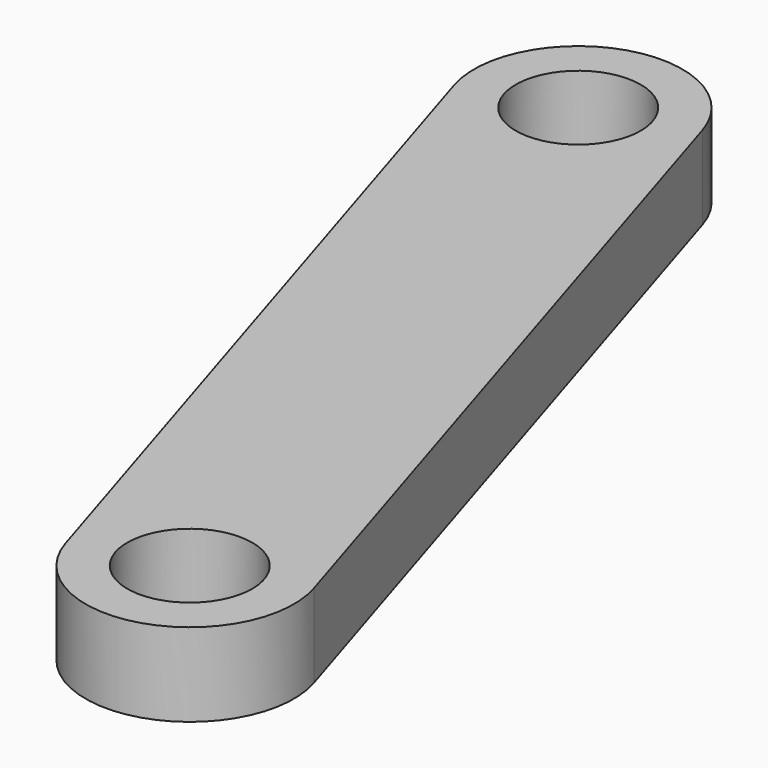
from build123d import *

# Parameters (mm, degrees)
F0_R     = 4.7625
F1_DEPTH = 6.35


# Not quite as in the source:
# - a feature names something its author has since deleted; it is built from what else it names


with BuildPart() as f1:
    # F0 (on Top) → F1 (new body)
    with BuildSketch(Plane.XY):
        with BuildLine():
            Line((7.5795164193, 2.3568701916), (-11.2418835807, 62.8850701916))
            ThreePointArc((-11.2418835807, 62.8850701916), (-21.1782701916, 68.1077164193), (-26.4009164193, 58.1713298084))
            Line((-26.4009164193, 58.1713298084), (-7.5795164193, -2.3568701916))
            ThreePointArc((-7.5795164193, -2.3568701916), (2.3568701916, -7.5795164193), (7.5795164193, 2.3568701916))
        make_face()
        Circle(F0_R, mode=Mode.SUBTRACT)
        with Locations((-18.8214, 60.5282)):
            Circle(F0_R, mode=Mode.SUBTRACT)
    extrude(amount=F1_DEPTH)


solid = f1.part
